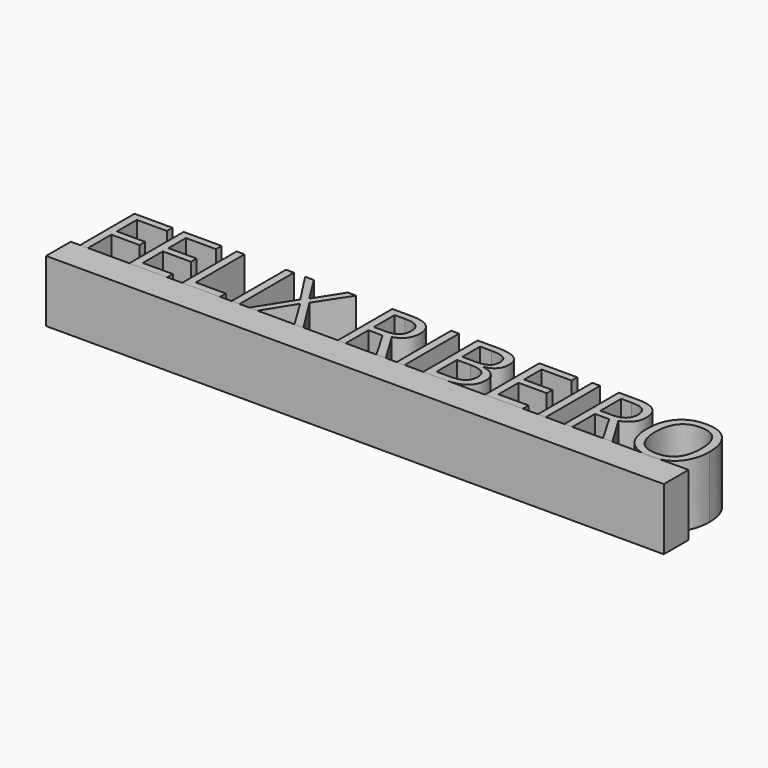
from build123d import *

# Parameters (mm, degrees)
F0_W         = 100
F0_H         = 5
F1_DEPTH     = 10
F2_TEXT_SIZE = 15.4142581888
F3_DEPTH     = 10


# Not quite as in the source:
# - Text() gives the source's letters only with a copy of the font that has no kerning and outlines rounded to 1/6400 em; it was checked with that copy


with BuildPart() as f1:
    # F0 (on Top) → F1 (new body)
    with BuildSketch(Plane.XY):
        with Locations((50, -2.5)):
            Rectangle(F0_W, F0_H)
    extrude(amount=F1_DEPTH)

    # F2 (on Top) → F3 (join)
    with BuildSketch(Plane.XY):
        with Locations((0, 0)):
            Text('FELIX RIBEIRO', F2_TEXT_SIZE, font='Open Sans', text_align=(TextAlign.LEFT, TextAlign.BOTTOM))
    extrude(amount=F3_DEPTH)


solid = f1.part
